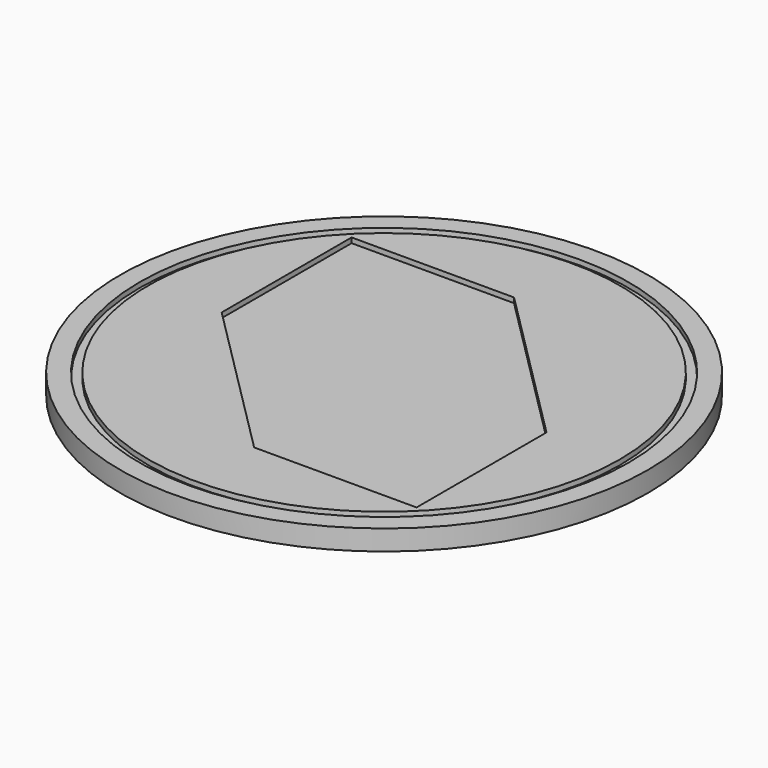
from build123d import *

# Parameters (mm, degrees)
F0_R     = 41.275
F1_DEPTH = 3.175
F2_R     = 38.2337964231
F2_R_2   = 36.8557965157
F3_DEPTH = 0.79375
F5_DEPTH = 0.79375


# Not quite as in the source:
# - a length typed as a fraction of an inch, garbled in the dataset ("3 / 203.2 mm" for 3/8 in), is restored


with BuildPart() as f1:
    # F0 (on Top) → F1 (new body)
    with BuildSketch(Plane.XY):
        Circle(F0_R)
    extrude(amount=F1_DEPTH)

    # F2 (on face) → F3 (cut)
    with BuildSketch(Plane.XY.offset(3.175)):
        Circle(F2_R)
        Circle(F2_R_2, mode=Mode.SUBTRACT)
    extrude(amount=-F3_DEPTH, mode=Mode.SUBTRACT)

    # F4 (on face) → F5 (cut)
    with BuildSketch(Plane.XY.offset(3.175)):
        Polygon((25.4, 0), (0, 25.4), (-25.4, 25.4), (-25.4, 0), (0, -25.4), (25.4, -25.4), align=None)
    extrude(amount=-F5_DEPTH, mode=Mode.SUBTRACT)


solid = f1.part
